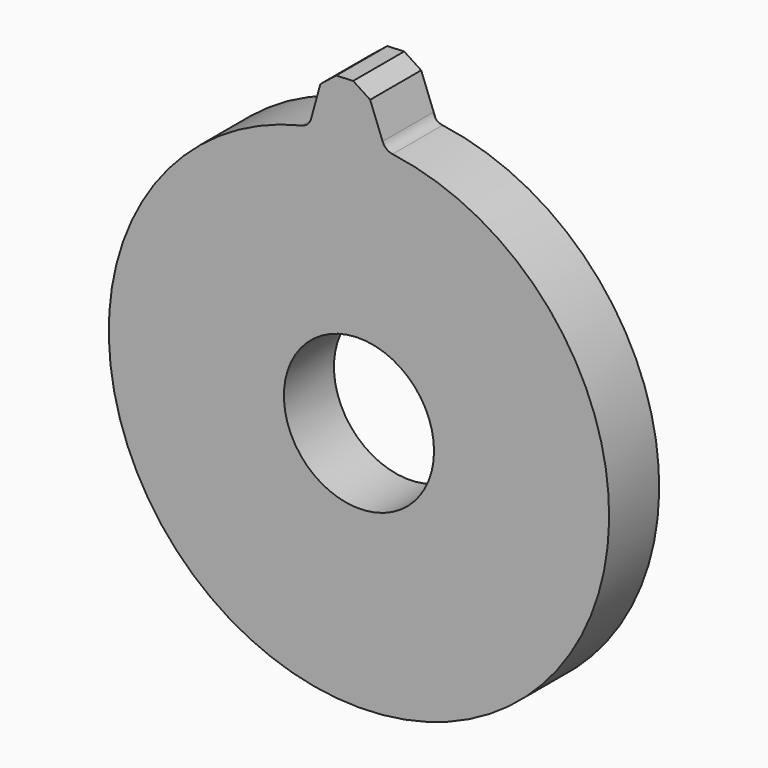
from build123d import *

# Parameters (mm, degrees)
F0_R     = 100
F1_DEPTH = 25
F3_DEPTH = 25.5
F4_SIZE  = 5
F5_R     = 5
F6_R     = 30
F7_DEPTH = 25.501


with BuildPart() as f1:
    # F0 (on Front) → F1 (new body)
    with BuildSketch(Plane.XZ):
        Circle(F0_R)
    extrude(amount=F1_DEPTH)

    # F2 (on face) → F3 (join)
    with BuildSketch(Plane.XZ.offset(25)):
        Polygon((-14.1001771265, 119.1687249449), (-19.9524563423, 97.9892825053), (10.5246777377, 99.4446135219), (2.6809251073, 119.9700489313), align=None)
    extrude(amount=-F3_DEPTH)

    # F4
    f4_edges = [f1.edges().sort_by_distance(p)[0] for p in [
        (2.680925, -12.25, 119.970049),
        (-14.100177, -12.25, 119.168725),
    ]]
    chamfer(f4_edges, length=F4_SIZE)

    # F5
    f5_edges = [f1.edges().sort_by_distance(p)[0] for p in [
        (-19.952456, -12.5, 97.989283),
        (10.524678, -12.5, 99.444614),
    ]]
    fillet(f5_edges, radius=F5_R)

    # F6 (on face) + F1_face1 (on face) → F7 (cut, through all)
    with BuildSketch(Plane.XZ.offset(25)):
        Circle(F6_R)
    with BuildSketch(Plane(origin=(0.0031470854, 0, -0.0659053797), x_dir=(1, 0, 0), z_dir=(0, 1, 0))):
        with BuildLine():
            ThreePointArc((13.4432882004, -99.1577485259), (4.7665750707, 99.8202786027), (-22.8304528013, -97.4256204252))
            ThreePointArc((-22.8304528013, -97.4256204252), (-20.5064145734, -98.6893061779), (-19.1524197717, -100.9619155688))
            Line((-19.1524197717, -100.9619155688), (-19.9556034276, -98.055187885))
            Line((-19.9556034276, -98.055187885), (10.5215306523, -99.5105189016))
            Line((10.5215306523, -99.5105189016), (9.4450314489, -102.3274887768))
            ThreePointArc((9.4450314489, -102.3274887768), (11.0094130673, -100.1942364433), (13.4432882004, -99.1577485259))
        make_face()
    extrude(amount=-F7_DEPTH, dir=(0, -1, 0), mode=Mode.SUBTRACT)


solid = f1.part
